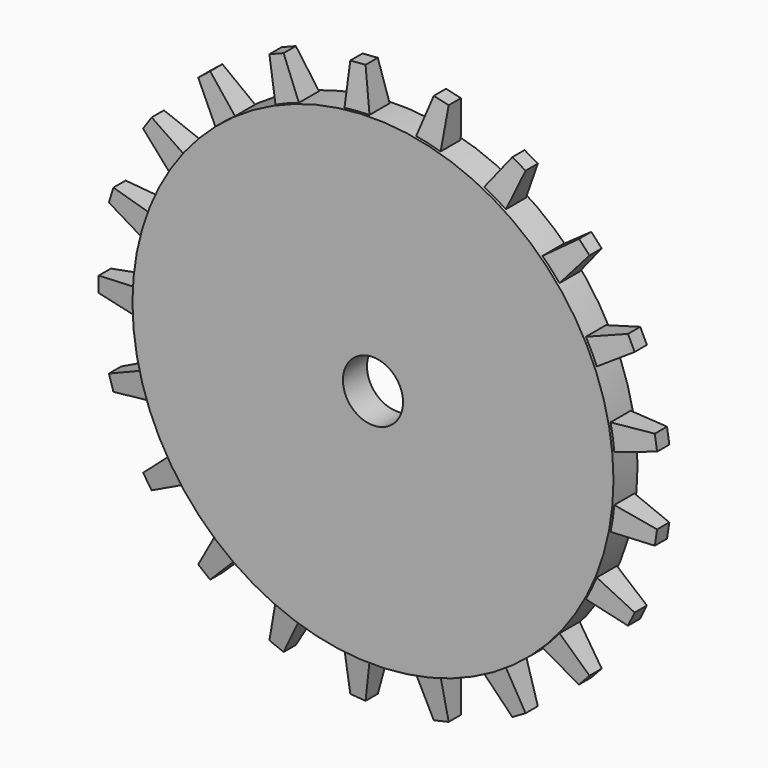
from build123d import *

# Parameters (mm, degrees)
F0_R     = 50.8
F0_R_2   = 6.35
F1_DEPTH = 6.35
F4_DEPTH = 12.7
F4_TAPER = 7
F6_COUNT = 21


# Not quite as in the source:
# - a feature names something its author has since deleted; it is built from what else it names


with BuildPart() as f1:
    # F0 (on Front) → F1 (new body)
    with BuildSketch(Plane.XZ):
        Circle(F0_R)
        Circle(F0_R_2, mode=Mode.SUBTRACT)
    extrude(amount=F1_DEPTH)

    # F3 (on offset) → F4 (join)
    with BuildSketch(Plane.YZ.offset(-46.482)):
        Polygon((-6.35, 3.175), (-6.35, 0), (-6.35, -3.175), (0, -3.175), (0, 3.175), align=None)
    extrude(amount=-F4_DEPTH, taper=F4_TAPER)

    # F6: F1 ×21 about axis
    f6_axis = Axis((0, -30.5892471224, 0), (0, -1, 0))


with BuildPart() as f1_1:
    add(f1.part)
    for i in range(1, F6_COUNT):
        add(f1.part.rotate(f6_axis, i * 360 / F6_COUNT))


solid = f1_1.part
